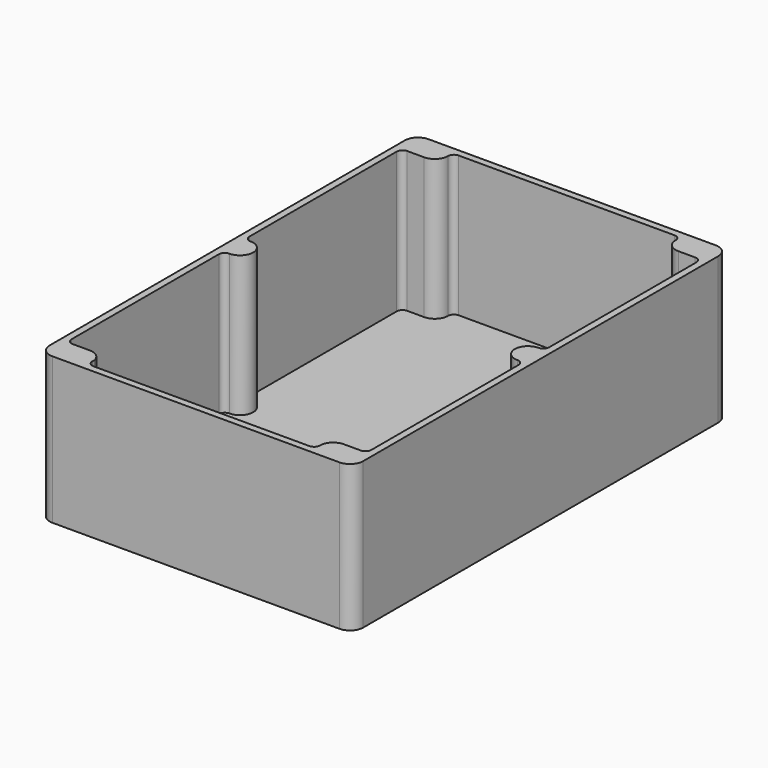
from build123d import *

# Parameters (mm, degrees)
F1_DEPTH = 3
F0_W     = 160
F0_H     = 240
F2_DEPTH = 74.8
F3_R     = 6.75
F4_R     = 2.99999


# Not quite as in the source:
# - a fillet or chamfer is up to 0.001 mm smaller than in the source, because OpenCascade refuses the exact size
# - ends of sketch curves that miss each other by under 0.0002 mm in the source are joined


with BuildPart() as f1:
    # F0 (on Top) → F1 (new body)
    with BuildSketch(Plane.XY):
        with BuildLine():
            Line((58.1, 113.45), (58.1, 116.5))
            Line((58.1, 116.5), (-58.1, 116.5))
            Line((-58.1, 116.5), (-58.1, 113.45))
            ThreePointArc((-58.1, 113.45), (-60.077029227, 108.677029227), (-64.85, 106.7))
            Line((-64.85, 106.7), (-76.5, 106.7))
            Line((-76.5, 106.7), (-76.5, 6.75))
            Line((-76.5, 6.75), (-73.5, 6.75))
            ThreePointArc((-73.5, 6.75), (-66.75, 0), (-73.5, -6.75))
            Line((-73.5, -6.75), (-76.5, -6.75))
            Line((-76.5, -6.75), (-76.5, -106.7))
            Line((-76.5, -106.7), (-64.7190213203, -106.7))
            ThreePointArc((-64.7190213203, -106.7), (-60.4393955388, -108.2301050614), (-58.1, -112.1267249867))
            Line((-58.1, -112.1267249867), (-58.1, -116.5))
            Line((-58.1, -116.5), (58.1, -116.5))
            Line((58.1, -116.5), (58.1, -113.45))
            ThreePointArc((58.1, -113.45), (60.077029227, -108.677029227), (64.85, -106.7))
            Line((64.85, -106.7), (76.5, -106.7))
            Line((76.5, -106.7), (76.5, -6.75))
            Line((76.5, -6.75), (73.5, -6.75))
            ThreePointArc((73.5, -6.75), (66.75, 0), (73.5, 6.75))
            Line((73.5, 6.75), (76.5, 6.75))
            Line((76.5, 6.75), (76.5, 106.7))
            Line((76.5, 106.7), (64.85, 106.7))
            ThreePointArc((64.85, 106.7), (60.077029227, 108.677029227), (58.1, 113.45))
        make_face()
    extrude(amount=F1_DEPTH)

    # F0 (on Top) → F2 (join)
    with BuildSketch(Plane.XY):
        Rectangle(F0_W, F0_H)
        Polygon((58.1, 116.5), (76.5, 116.5), (76.5, 106.7), (76.5, 6.75), (76.5, -6.75), (76.5, -106.7), (76.5, -116.5), (58.1, -116.5), (-58.1, -116.5), (-76.5, -116.5), (-76.5, -106.7), (-76.5, -6.75), (-76.5, 6.75), (-76.5, 106.7), (-76.5, 116.5), (-58.1, 116.5), align=None, mode=Mode.SUBTRACT)
        with BuildLine():
            Line((-58.1, 113.45), (-58.1, 116.5))
            Line((-58.1, 116.5), (-76.5, 116.5))
            Line((-76.5, 116.5), (-76.5, 106.7))
            Line((-76.5, 106.7), (-64.85, 106.7))
            ThreePointArc((-64.85, 106.7), (-60.077029227, 108.677029227), (-58.1, 113.45))
        make_face()
        with BuildLine():
            Line((76.5, 106.7), (76.5, 116.5))
            Line((76.5, 116.5), (58.1, 116.5))
            Line((58.1, 116.5), (58.1, 113.45))
            ThreePointArc((58.1, 113.45), (60.077029227, 108.677029227), (64.85, 106.7))
            Line((64.85, 106.7), (76.5, 106.7))
        make_face()
        with BuildLine():
            Line((-73.5, 6.75), (-76.5, 6.75))
            Line((-76.5, 6.75), (-76.5, -6.75))
            Line((-76.5, -6.75), (-73.5, -6.75))
            ThreePointArc((-73.5, -6.75), (-66.75, 0), (-73.5, 6.75))
        make_face()
        with BuildLine():
            Line((76.5, -6.75), (76.5, 6.75))
            Line((76.5, 6.75), (73.5, 6.75))
            ThreePointArc((73.5, 6.75), (66.75, 0), (73.5, -6.75))
            Line((73.5, -6.75), (76.5, -6.75))
        make_face()
        with BuildLine():
            Line((-64.7190213203, -106.7), (-76.5, -106.7))
            Line((-76.5, -106.7), (-76.5, -116.5))
            Line((-76.5, -116.5), (-58.1, -116.5))
            Line((-58.1, -116.5), (-58.1, -112.1267249867))
            ThreePointArc((-58.1, -112.1267249867), (-60.4393955388, -108.2301050614), (-64.7190213203, -106.7))
        make_face()
        with BuildLine():
            Line((76.5, -116.5), (76.5, -106.7))
            Line((76.5, -106.7), (64.85, -106.7))
            ThreePointArc((64.85, -106.7), (60.077029227, -108.677029227), (58.1, -113.45))
            Line((58.1, -113.45), (58.1, -116.500006485))
            Line((58.1, -116.500006485), (76.5, -116.5))
        make_face()
    extrude(amount=F2_DEPTH)

    # F3
    f3_edges = [f1.edges().sort_by_distance(p)[0] for p in [
        (80, 120, 37.4),
        (-80, 120, 37.4),
        (-80, -120, 37.4),
        (80, -120, 37.4),
    ]]
    fillet(f3_edges, radius=F3_R)

    # F4 (radius 3 in the source; OpenCascade refuses exactly that, so slightly less here)
    f4_edges = [f1.edges().sort_by_distance(p)[0] for p in [
        (-76.5, 106.7, 38.9),
        (-58.1, 116.5, 38.9),
        (-76.5, -6.75, 38.9),
        (58.1, 116.5, 38.9),
        (76.5, 106.7, 38.9),
        (76.5, -6.75, 38.9),
        (-76.5, 6.75, 38.9),
        (-76.5, -106.7, 38.9),
        (-58.1, -116.5, 38.9),
        (76.5, 6.75, 38.9),
        (76.5, -106.7, 38.9),
        (58.1, -116.5, 38.9),
    ]]
    fillet(f4_edges, radius=F4_R)


solid = f1.part
